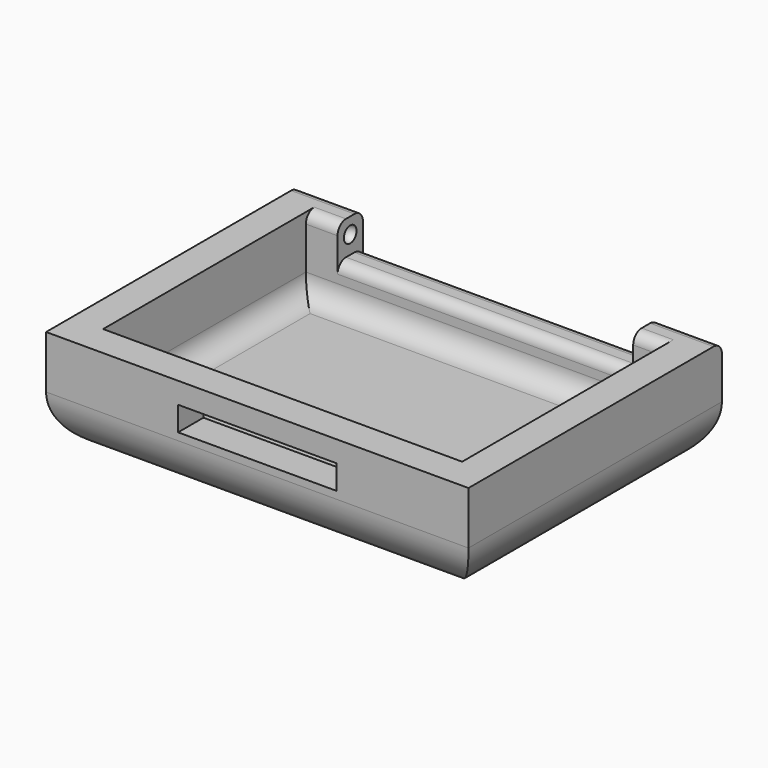
from build123d import *

# Parameters (mm, degrees)
F0_W      = 40
F0_H      = 30
F1_DEPTH  = 10
F2_R      = 5
F3_T      = -3
F4_W      = 28
F4_H      = 3
F5_DEPTH  = 3
F6_W      = 32.3581136763
F6_H      = 60.2468792349
F7_DEPTH  = 25
F8_R      = 0.75
F9_DEPTH  = 0.75
F10_R     = 0.74999
F11_W     = 14
F11_H     = 3
F12_DEPTH = 0.2
F13_R     = 1
F15_W     = 15
F15_H     = 2.3
F16_DEPTH = 3


# Not quite as in the source:
# - a fillet or chamfer is up to 0.001 mm smaller than in the source, because OpenCascade refuses the exact size


with BuildPart() as f1:
    # F0 (on Top) → F1 (new body)
    with BuildSketch(Plane.XY):
        Rectangle(F0_W, F0_H)
    extrude(amount=-F1_DEPTH)

    # F2
    f2_edges = [f1.edges().sort_by_distance(p)[0] for p in [
        (20, 0, -10),
        (0, 15, -10),
        (-20, 0, -10),
        (0, -15, -10),
    ]]
    fillet(f2_edges, radius=F2_R)

    # F3
    f3_openings = [f1.faces().sort_by_distance(p)[0] for p in [
        (0, 0, 0),
    ]]
    offset(amount=F3_T, openings=f3_openings)

    # F4 (on face) → F5 (cut)
    with BuildSketch(Plane.XY):
        with Locations((0, 13.5)):
            Rectangle(F4_W, F4_H)
    extrude(amount=-F5_DEPTH, mode=Mode.SUBTRACT)

    # F6 (on Top) → F7 (cut)
    with BuildSketch(Plane.XY):
        with Locations((16.1790568382, -2.0559011027)):
            Rectangle(F6_W, F6_H)
    extrude(amount=-F7_DEPTH, mode=Mode.SUBTRACT)

    # F8 (on face) → F9 (cut)
    with BuildSketch(Plane.YZ.offset(-14)):
        with Locations((13.5, -1.5)):
            Circle(F8_R)
    extrude(amount=-F9_DEPTH, mode=Mode.SUBTRACT)

    # F10 (radius 0.75 in the source; OpenCascade refuses exactly that, so slightly less here)
    f10_edges = [f1.edges().sort_by_distance(p)[0] for p in [
        (-14.75, 12.75, -1.5),
    ]]
    fillet(f10_edges, radius=F10_R)

    # F11 (on face) → F12 (cut)
    with BuildSketch(Plane.XY.offset(-3)):
        with Locations((-7, 13.5)):
            Rectangle(F11_W, F11_H)
    extrude(amount=-F12_DEPTH, mode=Mode.SUBTRACT)

    # F13
    f13_edges = [f1.edges().sort_by_distance(p)[0] for p in [
        (-17, 15, 0),
        (-15.5, 12, 0),
        (-7, 15, -3.2),
        (-7, 12, -3.2),
    ]]
    fillet(f13_edges, radius=F13_R)

    # F14: F1 across plane


with BuildPart() as f1_1:
    add(f1.part)
    add(f1.part.mirror(Plane.YZ))

    # F15 (on face) → F16 (cut, through all)
    with BuildSketch(Plane.XZ.offset(15)):
        with Locations((0, -3.15)):
            Rectangle(F15_W, F15_H)
    extrude(amount=-F16_DEPTH, mode=Mode.SUBTRACT)


solid = f1_1.part
